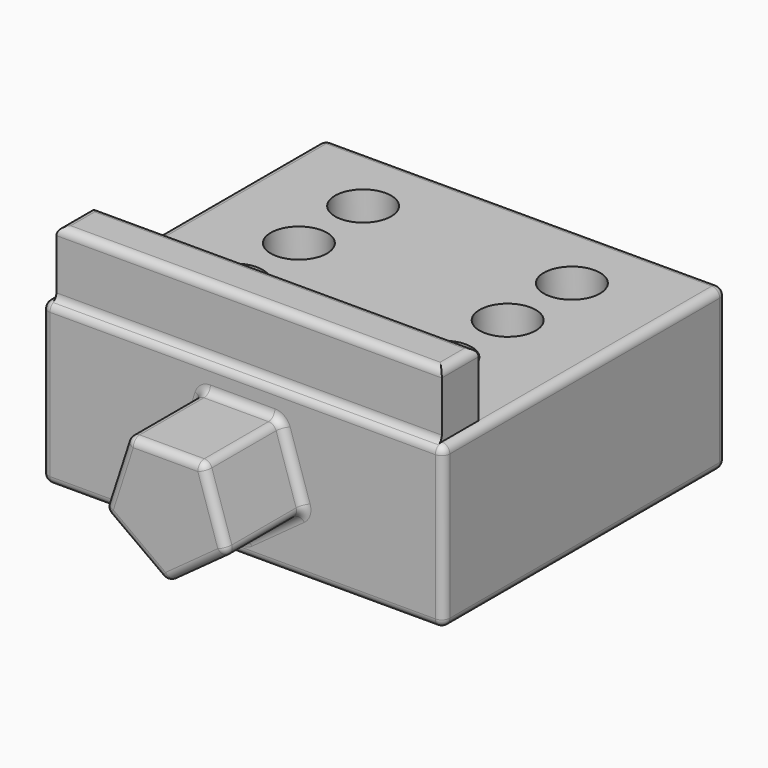
from build123d import *

# Parameters (mm, degrees)
F0_W        = 250
F0_H        = 100
F1_DEPTH    = 220
F2_R        = 5
F4_DEPTH    = 60
F5_W        = 240
F5_H        = 28.5892599821
F6_DEPTH    = 40
F7_T1_DEPTH = 240
F7_T3_DEPTH = 265
F7_T5_DEPTH = 53.5892599821
F8_R        = 5
F9_R        = 17.5
F10_DEPTH   = 20


# Not quite as in the source:
# - a fillet or chamfer that OpenCascade refuses, or shapes differently, is made with other operations: its cross-section is extruded or revolved along the edge and cut away or added


with BuildPart() as f1:
    # F0 (on Front) → F1 (new body)
    with BuildSketch(Plane.XZ):
        Rectangle(F0_W, F0_H)
    extrude(amount=F1_DEPTH)

    # F2
    f2_edges = [f1.edges().sort_by_distance(p)[0] for p in [
        (125, -110, 50),
        (-125, -110, 50),
        (0, 0, 50),
        (0, -220, 50),
        (-125, -110, -50),
        (125, -110, -50),
        (0, 0, -50),
        (0, -220, -50),
        (125, -220, 0),
        (-125, -220, 0),
        (-125, 0, 0),
        (125, 0, 0),
    ]]
    fillet(f2_edges, radius=F2_R)

    # F3 (on face) → F4 (join)
    with BuildSketch(Plane.XZ.offset(220)):
        Polygon((23.7203992628, 32.6483286917), (-23.7203992628, 32.6483286917), (-38.380412234, -12.4705518844), (0, -40.3555536147), (38.380412234, -12.4705518844), align=None)
    extrude(amount=F4_DEPTH)

    # F5 (on face) → F6 (join)
    with BuildSketch(Plane.XY.offset(50)):
        with Locations((0, -200.7053700089)):
            Rectangle(F5_W, F5_H)
    extrude(amount=F6_DEPTH)

    # F7: fillet of radius 5 on 6 edges, made by hand

    # F7_s2 → F7_t1 (join)
    with BuildSketch(Plane.YZ.offset(-120)):
        with BuildLine():
            ThreePointArc((-217.5, 49.3301270189), (-215.6698729811, 51.1602540378), (-215, 53.6602540378))
            Line((-215, 53.6602540378), (-215, 50))
            ThreePointArc((-215, 50), (-216.2940952255, 49.8296291314), (-217.5, 49.3301270189))
        make_face()
    extrude(amount=F7_T1_DEPTH)

    # F7_s4 → F7_t3 (cut)
    with BuildSketch(Plane.YZ.offset(-132.5)):
        with BuildLine():
            ThreePointArc((-186.4107400179, 85), (-187.875206112, 88.5355339059), (-191.4107400179, 90))
            Line((-191.4107400179, 90), (-186.4107400179, 90))
            Line((-186.4107400179, 90), (-186.4107400179, 85))
        make_face()
        with BuildLine():
            ThreePointArc((-215, 85), (-213.5355339059, 88.5355339059), (-210, 90))
            Line((-210, 90), (-215, 90))
            Line((-215, 90), (-215, 85))
        make_face()
    extrude(amount=F7_T3_DEPTH, mode=Mode.SUBTRACT)

    # F7_s6 → F7_t5 (cut)
    with BuildSketch(Plane.XZ.offset(173.9107400179)):
        with BuildLine():
            ThreePointArc((-120, 85), (-118.5355339059, 88.5355339059), (-115, 90))
            Line((-115, 90), (-120, 90))
            Line((-120, 90), (-120, 85))
        make_face()
        with BuildLine():
            ThreePointArc((120, 85), (118.5355339059, 88.5355339059), (115, 90))
            Line((115, 90), (120, 90))
            Line((120, 90), (120, 85))
        make_face()
    extrude(amount=F7_T5_DEPTH, mode=Mode.SUBTRACT)

    # F8
    f8_edges = [f1.edges().sort_by_distance(p)[0] for p in [
        (0, -220, 32.648329),
        (31.050406, -220, 10.088888),
        (19.190206, -220, -26.413053),
        (-19.190206, -220, -26.413053),
        (-31.050406, -220, 10.088888),
        (31.050406, -280, 10.088888),
        (0, -280, 32.648329),
        (-31.050406, -280, 10.088888),
        (-19.190206, -280, -26.413053),
        (19.190206, -280, -26.413053),
        (-23.720399, -250, 32.648329),
        (23.720399, -250, 32.648329),
        (38.380412, -250, -12.470552),
        (0, -250, -40.355554),
        (-38.380412, -250, -12.470552),
    ]]
    fillet(f8_edges, radius=F8_R)

    # F9 (on face) → F10 (cut)
    with BuildSketch(Plane.XY.offset(50)):
        with Locations((-65, -45)):
            Circle(F9_R)
        with Locations((-65, -95)):
            Circle(F9_R)
        with Locations((-65, -145)):
            Circle(F9_R)
        with Locations((65, -145)):
            Circle(F9_R)
        with Locations((65, -95)):
            Circle(F9_R)
        with Locations((65, -45)):
            Circle(F9_R)
    extrude(amount=-F10_DEPTH, mode=Mode.SUBTRACT)


solid = f1.part
